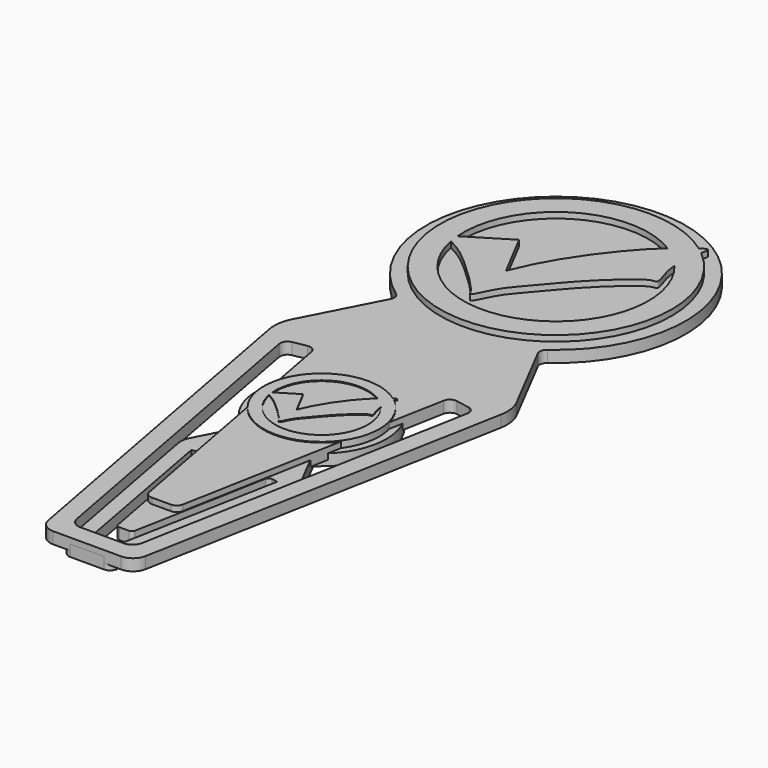
from build123d import *

# Parameters (mm, degrees)
F1_DEPTH      = 0.79375
F3_DEPTH      = 0.396875
F4_R          = 7.9375
F4_R_2        = 6.35
F5_DEPTH      = 0.396875
F6_SCALE      = 0.5
F7_DEPTH      = 0.381
F9_DEPTH      = 0.396875
F9_DEPTH_BACK = 0.381
F10_DEPTH     = 0.254


with BuildPart() as f1:
    # F0 (on Top) → F1 (new body)
    with BuildSketch(Plane.XY):
        with BuildLine():
            Line((-2.3309670021, 0), (0, 0))
            Line((0, 0), (2.3309670021, 0))
            ThreePointArc((2.3309670021, 0), (2.9801980228, 0.2344917904), (3.3297452947, 0.8297262171))
            Line((3.3297452947, 0.8297262171), (7.9402363107, 25.5506411715))
            ThreePointArc((7.9402363107, 25.5506411715), (7.956177787, 26.3864578765), (7.6999208348, 27.1821814902))
            Line((7.6999208348, 27.1821814902), (5.0455684503, 32.3199451691))
            ThreePointArc((5.0455684503, 32.3199451691), (5.0028082613, 32.6711959216), (5.199765069, 32.9651577232))
            ThreePointArc((5.199765069, 32.9651577232), (0, 49.0658819052), (-5.199765069, 32.9651577232))
            ThreePointArc((-5.199765069, 32.9651577232), (-5.0028082613, 32.6711959216), (-5.0455684503, 32.3199451691))
            Line((-5.0455684503, 32.3199451691), (-7.6999208348, 27.1821814902))
            ThreePointArc((-7.6999208348, 27.1821814902), (-7.956177787, 26.3864578765), (-7.9402363107, 25.5506411715))
            Line((-7.9402363107, 25.5506411715), (-3.3297452947, 0.8297262171))
            ThreePointArc((-3.3297452947, 0.8297262171), (-2.9801980228, 0.2344917904), (-2.3309670021, 0))
        make_face()
        with BuildLine():
            Line((1.4869340041, 1.27), (0, 1.27))
            Line((0, 1.27), (-1.4869340041, 1.27))
            ThreePointArc((-1.4869340041, 1.27), (-1.9738572697, 1.4458688428), (-2.2360177236, 1.8922946628))
            Line((-2.2360177236, 1.8922946628), (-6.4569152141, 24.5242545847))
            ThreePointArc((-6.4569152141, 24.5242545847), (-6.3765052472, 24.9046552004), (-6.0506629593, 25.1167806224))
            Line((-6.0506629593, 25.1167806224), (-5.1238263569, 25.2896371626))
            ThreePointArc((-5.1238263569, 25.2896371626), (-4.7434257411, 25.2092271956), (-4.5313003191, 24.8833849078))
            Line((-4.5313003191, 24.8833849078), (-1.1521664103, 6.7648631086))
            ThreePointArc((-1.1521664103, 6.7648631086), (-0.9773927744, 6.4672458952), (-0.652777264, 6.35))
            Line((-0.652777264, 6.35), (0, 6.35))
            Line((0, 6.35), (0.652777264, 6.35))
            ThreePointArc((0.652777264, 6.35), (0.9773927744, 6.4672458952), (1.1521664103, 6.7648631086))
            Line((1.1521664103, 6.7648631086), (4.5313003191, 24.8833849078))
            ThreePointArc((4.5313003191, 24.8833849078), (4.7434257411, 25.2092271956), (5.1238263569, 25.2896371626))
            Line((5.1238263569, 25.2896371626), (6.0506629593, 25.1167806224))
            ThreePointArc((6.0506629593, 25.1167806224), (6.3765052472, 24.9046552004), (6.4569152141, 24.5242545847))
            Line((6.4569152141, 24.5242545847), (2.2360177236, 1.8922946628))
            ThreePointArc((2.2360177236, 1.8922946628), (1.9738572697, 1.4458688428), (1.4869340041, 1.27))
        make_face(mode=Mode.SUBTRACT)
    extrude(amount=F1_DEPTH)

    # F2 (on face) → F3 (join)
    with BuildSketch(Plane.XY.offset(0.79375)):
        with BuildLine():
            Line((-1.7935041105, 38.1308123469), (-3.4859369043, 41.377518326))
            Line((-3.4859369043, 41.377518326), (-6.8725775927, 39.3059626222))
            add(Edge.make_bspline(
                [(-1.7935041105, 38.1308123469), (-1.5460361909, 38.7222766807), (-0.9971508849, 40.0341480633), (0.5953097014, 42.5597733053), (2.2310910127, 44.5105527375), (3.3913678773, 45.6923635738), (5.3435102325, 47.1937213559), (5.0136861896, 46.1807991461), (4.8408650471, 44.6126122533), (4.9430262636, 43.4406367652), (5.4785201607, 42.1002420808), (4.8811005333, 42.2492470038), (3.2298156355, 40.8818535801), (1.5724000209, 39.174477809), (0.299282713, 37.5554763055), (-0.8991247807, 36.3094405174), (-1.5581280156, 34.5693359881), (-1.7969462491, 35.2766666209), (-3.3825302975, 36.8205235473), (-4.6992028179, 38.0075509587), (-5.5275763145, 38.6082155164), (-6.3937390324, 39.05755526), (-6.8725775927, 39.3059626222)],
                knots=[0, 0, 0, 0, 0.0571741991, 0.126812711, 0.19008784, 0.2457649115, 0.2996259061, 0.3285078729, 0.3800178056, 0.426690923, 0.4690787439, 0.4912517254, 0.5483271022, 0.6125144728, 0.669296969, 0.7247630586, 0.7721811152, 0.7957724037, 0.8563127526, 0.910840938, 0.9507104196, 1, 1, 1, 1], degree=3))
        make_face()
    extrude(amount=F3_DEPTH)

    # F4 (on face) → F5 (join)
    with BuildSketch(Plane.XY.offset(0.79375)):
        with Locations((0, 40.1758819052)):
            Circle(F4_R)
        with Locations((0, 40.1758819052)):
            Circle(F4_R_2, mode=Mode.SUBTRACT)
    extrude(amount=F5_DEPTH)


with BuildPart() as f6_1:
    # F6: copy of F1
    add(f1.part.scale(F6_SCALE))

    # F7 (add): a face of the model
    f7_faces = [f6_1.faces().sort_by_distance(p)[0] for p in [
        (0, 14.787590063, 0),
    ]]
    extrude(f7_faces, amount=F7_DEPTH)

    # F8 (on Top) → F9 (join, two sides)
    with BuildSketch(Plane.XY) as f9_sk:
        with BuildLine():
            Line((-0.8179266392, 1.2058972601), (-2.9330298855, 12.6638541183))
            Line((-2.9330298855, 12.6638541183), (-3.308619095, 12.5998717327))
            Line((-3.308619095, 12.5998717327), (-1.0899560502, 0.5809097763))
            Line((-1.0899560502, 0.5809097763), (1.0681329547, 0.5809097763))
            Line((1.0681329547, 0.5809097763), (3.3495018724, 12.5284111127))
            Line((3.3495018724, 12.5284111127), (2.9752634728, 12.5998717327))
            Line((2.9752634728, 12.5998717327), (0.7992977101, 1.2043654401))
            ThreePointArc((0.7992977101, 1.2043654401), (0.7116932675, 1.0562807082), (0.5498054436, 0.9980058535))
            Line((0.5498054436, 0.9980058535), (-0.5681467409, 0.9980058535))
            ThreePointArc((-0.5681467409, 0.9980058535), (-0.7306343054, 1.0567783161), (-0.8179266392, 1.2058972601))
        make_face()
    extrude(amount=F9_DEPTH)
    extrude(f9_sk.sketch, amount=-F9_DEPTH_BACK)

    # F10 (add): a face of the model
    f10_faces = [f6_1.faces().sort_by_distance(p)[0] for p in [
        (-0.0188035912, 20.1025580514, 0.5953125),
    ]]
    extrude(f10_faces, amount=F10_DEPTH)


solid = Compound([f1.part, f6_1.part])
